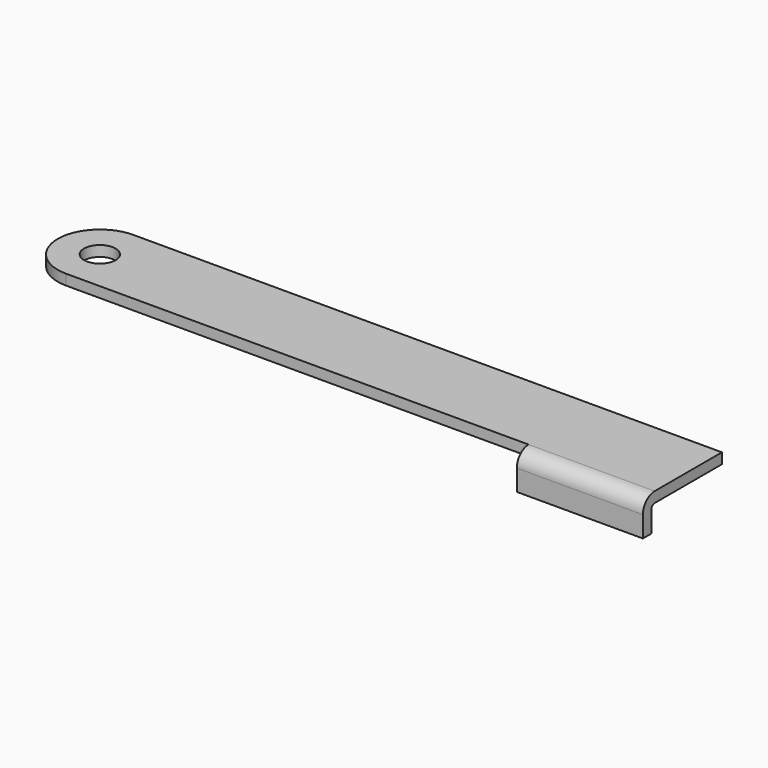
from build123d import *

# Parameters (mm, degrees)
F0_W     = 150
F0_H     = 20
F1_DEPTH = 2.5
F3_D     = 7.5
F4_R     = 9.99999
F5_W     = 2.5
F5_H     = 5
F6_DEPTH = 30


# Not quite as in the source:
# - a fillet or chamfer is up to 0.001 mm smaller than in the source, because OpenCascade refuses the exact size


with BuildPart() as f1:
    # F0 (on Top) → F1 (new body)
    with BuildSketch(Plane.XY):
        Rectangle(F0_W, F0_H)
    extrude(amount=F1_DEPTH)

    # F3 (through all)
    with Locations(Plane.XY.offset(2.5)):
        with Locations((-65, 0)):
            Hole(F3_D / 2)

    # F4 (radius 10 in the source; OpenCascade refuses exactly that, so slightly less here)
    f4_edges = [f1.edges().sort_by_distance(p)[0] for p in [
        (-75, -10, 1.25),
        (-75, 10, 1.25),
    ]]
    fillet(f4_edges, radius=F4_R)

    # F5 (on face) → F6 (join)
    with BuildSketch(Plane.YZ.offset(75)):
        with BuildLine():
            Line((-10, 0), (-10, 2.5))
            ThreePointArc((-10, 2.5), (-12.4748737342, 1.4748737342), (-13.5, -1))
            Line((-13.5, -1), (-11, -1))
            ThreePointArc((-11, -1), (-10.7071067812, -0.2928932188), (-10, 0))
        make_face()
        with Locations((-12.25, -3.5)):
            Rectangle(F5_W, F5_H)
    extrude(amount=-F6_DEPTH)


solid = f1.part
